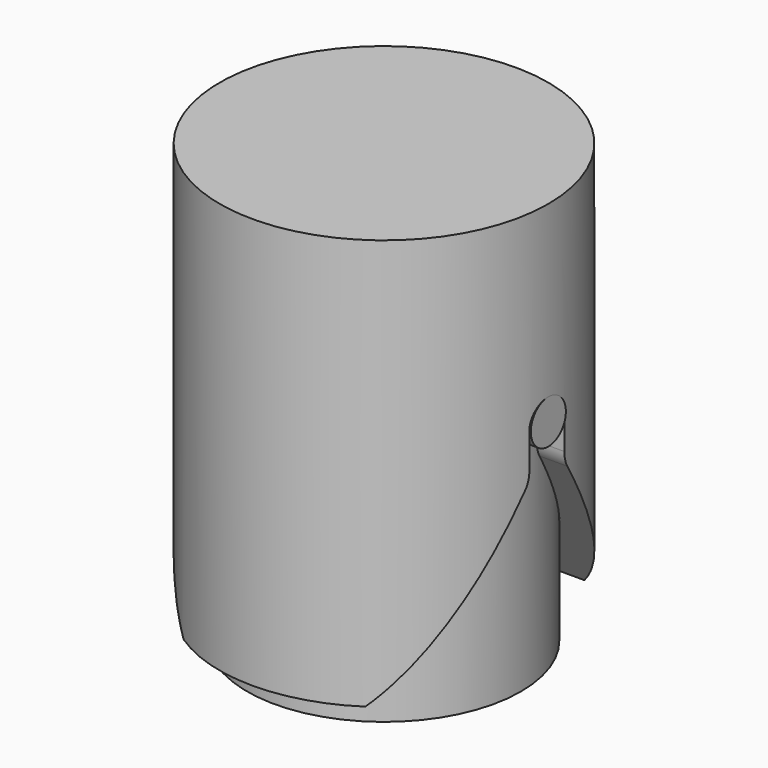
from build123d import *

# Parameters (mm, degrees)
F0_R      = 25
F0_R_2    = 20
F1_DEPTH  = 35
F0_R_3    = 3.5
F0_R_4    = 2.5
F2_DEPTH  = 25
F3_DEPTH  = 25
F5_R      = 4
F6_DEPTH  = 10
F8_R      = 20
F8_R_2    = 3.5
F9_DEPTH  = 30
F10_R     = 20
F11_DEPTH = 15
F12_R     = 30
F12_R_2   = 25
F12_R_3   = 20
F13_DEPTH = 5
F14_DEPTH = 70
F16_DEPTH = 100
F19_DEPTH = 25
F21_DEPTH = 30


with BuildPart() as f1:
    # F0 (on Top) → F1 (new body)
    with BuildSketch(Plane.XY):
        Circle(F0_R)
        Circle(F0_R_2, mode=Mode.SUBTRACT)
    extrude(amount=F1_DEPTH)

    # F0 (on Top) → F2 (join)
    with BuildSketch(Plane.XY):
        Circle(F0_R)
        Circle(F0_R_2, mode=Mode.SUBTRACT)
        Circle(F0_R_2)
        with Locations((-8.4852813742, -8.4852813742)):
            Circle(F0_R_3, mode=Mode.SUBTRACT)
        with Locations((8.4852813742, -8.4852813742)):
            Circle(F0_R_3, mode=Mode.SUBTRACT)
        with Locations((-11.0865543901, 4.5922011884)):
            Circle(F0_R_3, mode=Mode.SUBTRACT)
        with Locations((11.0865543901, 4.5922011884)):
            Circle(F0_R_3, mode=Mode.SUBTRACT)
        with Locations((0, 12)):
            Circle(F0_R_3, mode=Mode.SUBTRACT)
        with Locations((-8.4852813742, -8.4852813742)):
            Circle(F0_R_3)
        with Locations((-8.4852813742, -8.4852813742)):
            Circle(F0_R_4, mode=Mode.SUBTRACT)
        with Locations((11.0865543901, 4.5922011884)):
            Circle(F0_R_3)
        with Locations((11.0865543901, 4.5922011884)):
            Circle(F0_R_4, mode=Mode.SUBTRACT)
        with Locations((8.4852813742, -8.4852813742)):
            Circle(F0_R_3)
        with Locations((8.4852813742, -8.4852813742)):
            Circle(F0_R_4, mode=Mode.SUBTRACT)
        with Locations((-11.0865543901, 4.5922011884)):
            Circle(F0_R_3)
        with Locations((-11.0865543901, 4.5922011884)):
            Circle(F0_R_4, mode=Mode.SUBTRACT)
        with Locations((0, 12)):
            Circle(F0_R_3)
        with Locations((0, 12)):
            Circle(F0_R_4, mode=Mode.SUBTRACT)
        with Locations((-8.4852813742, -8.4852813742)):
            Circle(F0_R_4)
        with Locations((-11.0865543901, 4.5922011884)):
            Circle(F0_R_4)
        with Locations((0, 12)):
            Circle(F0_R_4)
        with Locations((11.0865543901, 4.5922011884)):
            Circle(F0_R_4)
        with Locations((8.4852813742, -8.4852813742)):
            Circle(F0_R_4)
    extrude(amount=-F2_DEPTH)

    # F0 (on Top) → F3 (join)
    with BuildSketch(Plane.XY):
        with Locations((0, 12)):
            Circle(F0_R_3)
        with Locations((0, 12)):
            Circle(F0_R_4, mode=Mode.SUBTRACT)
        with Locations((-11.0865543901, 4.5922011884)):
            Circle(F0_R_3)
        with Locations((-11.0865543901, 4.5922011884)):
            Circle(F0_R_4, mode=Mode.SUBTRACT)
        with Locations((11.0865543901, 4.5922011884)):
            Circle(F0_R_3)
        with Locations((11.0865543901, 4.5922011884)):
            Circle(F0_R_4, mode=Mode.SUBTRACT)
        with Locations((8.4852813742, -8.4852813742)):
            Circle(F0_R_3)
        with Locations((8.4852813742, -8.4852813742)):
            Circle(F0_R_4, mode=Mode.SUBTRACT)
        with Locations((-8.4852813742, -8.4852813742)):
            Circle(F0_R_3)
        with Locations((-8.4852813742, -8.4852813742)):
            Circle(F0_R_4, mode=Mode.SUBTRACT)
    extrude(amount=F3_DEPTH)

    # F5 (on offset) → F6 (join)
    with BuildSketch(Plane.YZ.offset(-20)):
        with Locations((0, 20)):
            Circle(F5_R)
    extrude(amount=-F6_DEPTH)

    # F7: F1 across plane


with BuildPart() as f1_1:
    add(f1.part)
    add(f1.part.mirror(Plane.YZ))


with BuildPart() as f9:
    # F8 (on Top) → F9 (new body)
    with BuildSketch(Plane.XY):
        Circle(F8_R)
        with Locations((-8.4852813742, -8.4852813742)):
            Circle(F8_R_2, mode=Mode.SUBTRACT)
        with Locations((8.4852813742, -8.4852813742)):
            Circle(F8_R_2, mode=Mode.SUBTRACT)
        with Locations((-11.0865543901, 4.5922011884)):
            Circle(F8_R_2, mode=Mode.SUBTRACT)
        with Locations((11.0865543901, 4.5922011884)):
            Circle(F8_R_2, mode=Mode.SUBTRACT)
        with Locations((0, 12)):
            Circle(F8_R_2, mode=Mode.SUBTRACT)
    extrude(amount=F9_DEPTH)



with BuildPart() as f9b:
    # F0 (on Top) → F9, piece 2 (new body)
    with BuildSketch(Plane.XY):
        with Locations((0, 12)):
            Circle(F0_R_4)
    extrude(amount=F9_DEPTH)


with BuildPart() as f9c:
    # F0 (on Top) → F9, piece 3 (new body)
    with BuildSketch(Plane.XY):
        with Locations((-11.0865543901, 4.5922011884)):
            Circle(F0_R_4)
    extrude(amount=F9_DEPTH)


with BuildPart() as f9d:
    # F0 (on Top) → F9, piece 4 (new body)
    with BuildSketch(Plane.XY):
        with Locations((-8.4852813742, -8.4852813742)):
            Circle(F0_R_4)
    extrude(amount=F9_DEPTH)


with BuildPart() as f9e:
    # F0 (on Top) → F9, piece 5 (new body)
    with BuildSketch(Plane.XY):
        with Locations((8.4852813742, -8.4852813742)):
            Circle(F0_R_4)
    extrude(amount=F9_DEPTH)


with BuildPart() as f9f:
    # F0 (on Top) → F9, piece 6 (new body)
    with BuildSketch(Plane.XY):
        with Locations((11.0865543901, 4.5922011884)):
            Circle(F0_R_4)
    extrude(amount=F9_DEPTH)


with BuildPart() as f9_1:
    add(f9.part)

    add(f9b.part)  # F11 merges F9b

    add(f9c.part)  # F11 merges F9c

    add(f9d.part)  # F11 merges F9d

    add(f9e.part)  # F11 merges F9e

    add(f9f.part)  # F11 merges F9f
    # F10 (on face) → F11 (join, symmetric)
    with BuildSketch(Plane.XY.offset(35)):
        Circle(F10_R)
    extrude(amount=F11_DEPTH, both=True)

    # F12 (on face) → F13 (join)
    with BuildSketch(Plane.XY.offset(50)):
        Circle(F12_R)
        Circle(F12_R_2, mode=Mode.SUBTRACT)
        Circle(F12_R_2)
        Circle(F12_R_3, mode=Mode.SUBTRACT)
        Circle(F12_R_3)
    extrude(amount=F13_DEPTH)

    # F12 (on face) → F14 (join)
    with BuildSketch(Plane.XY.offset(50)):
        Circle(F12_R)
        Circle(F12_R_2, mode=Mode.SUBTRACT)
    extrude(amount=-F14_DEPTH)

    # F15 (on offset) → F16 (cut)
    with BuildSketch(Plane.YZ.offset(-20)):
        with BuildLine():
            Line((4, 13.4941234329), (4, 20))
            ThreePointArc((4, 20), (0, 24), (-4, 20))
            Line((-4, 20), (-4, 13.4941234329))
            ThreePointArc((-4, 13.4941234329), (-4.2093216675, 12.0625504817), (-4.8197604458, 10.7508412254))
            Line((-4.8197604458, 10.7508412254), (-25, -20))
            Line((-25, -20), (25, -20))
            Line((25, -20), (4.8197604458, 10.7508412254))
            ThreePointArc((4.8197604458, 10.7508412254), (4.2093216675, 12.0625504817), (4, 13.4941234329))
        make_face()
    extrude(amount=-F16_DEPTH, mode=Mode.SUBTRACT)

    # F18 (on offset) → F19 (cut)
    with BuildSketch(Plane.YZ.offset(20)):
        with BuildLine():
            Line((4, 13.4941234329), (4, 20))
            ThreePointArc((4, 20), (0, 24), (-4, 20))
            Line((-4, 20), (-4, 13.4941234329))
            ThreePointArc((-4, 13.4941234329), (-4.2093216675, 12.0625504817), (-4.8197604458, 10.7508412254))
            Line((-4.8197604458, 10.7508412254), (-25, -20))
            Line((-25, -20), (25, -20))
            Line((25, -20), (4.8197604458, 10.7508412254))
            ThreePointArc((4.8197604458, 10.7508412254), (4.2093216675, 12.0625504817), (4, 13.4941234329))
        make_face()
    extrude(amount=F19_DEPTH, mode=Mode.SUBTRACT)

    # F20 (on Right) → F21 (cut, symmetric)
    with BuildSketch(Plane.YZ):
        Polygon((-14.5, -4), (-25, -20), (25, -20), (14.5, -4), align=None)
    extrude(amount=F21_DEPTH, both=True, mode=Mode.SUBTRACT)


solid = Compound([f1_1.part, f9_1.part])
